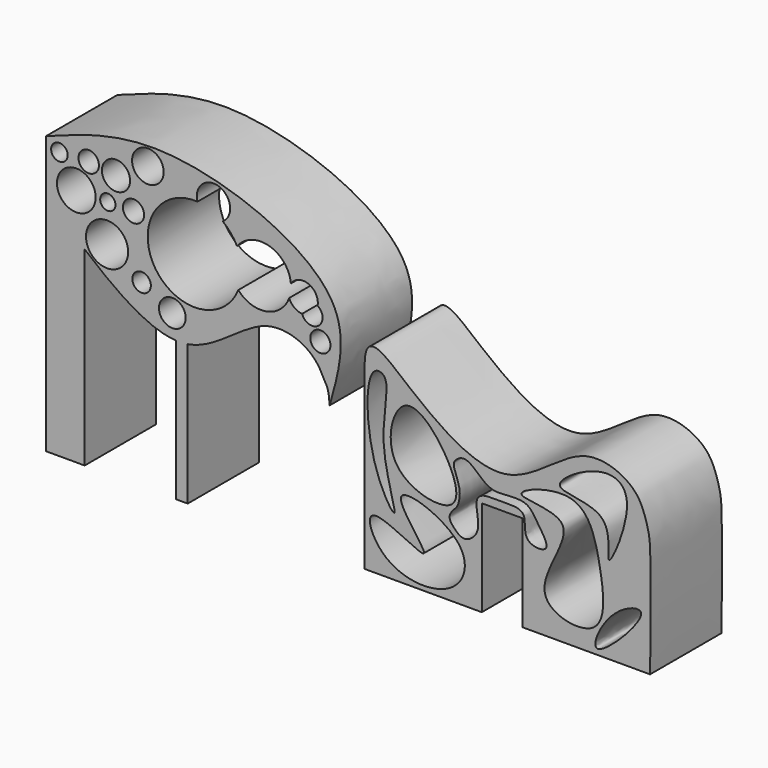
from build123d import *

# Parameters (mm, degrees)
F1_DEPTH = 25
F0_R     = 3.7468792803
F0_R_2   = 2.5930177145
F0_R_3   = 5.9129187482
F0_R_4   = 2.8310435697
F0_R_5   = 5.4292359739
F0_R_6   = 2.1382808776
F0_R_7   = 2.3192836327
F0_R_8   = 3.9494993962
F0_R_9   = 2.868756134
F0_R_10  = 2.9701337928
F0_R_11  = 4.4308880969
F2_DEPTH = 25
F3_DEPTH = 25


# Not quite as in the source:
# - a feature names something its author has since deleted; it is built from what else it names


with BuildPart() as f1:
    # F0 (on Front) → F1 (new body)
    with BuildSketch(Plane.XZ):
        with BuildLine():
            Line((0, 50.3192950504), (0, 0))
            Line((0, 0), (32.8370295465, 0))
            Line((32.8370295465, 0), (32.8370295465, 26.8986206502))
            Line((32.8370295465, 26.8986206502), (44.2832522094, 26.8986206502))
            Line((44.2832522094, 26.8986206502), (44.2832522094, 0))
            Line((44.2832522094, 0), (80.0090666652, 0))
            add(Edge.make_bspline(
                [(0, 50.3192950504), (0, 59.5670401082), (14.3941760892, 46.8630363864), (39.6650361306, 28.0602790595), (59.9123084229, 52.1391667117), (75.1310389197, 45.7993651518), (78.2880633586, 39.9618765746), (79.9116639555, 34.1838305265), (80.0826767357, 30.1384767337), (80.1342161447, 27.1190199724), (80.2397243312, 10.6725007615), (80.0090666652, 0)],
                knots=[0, 0, 0, 0, 0.1048673687, 0.2855122378, 0.4444928656, 0.5600818488, 0.6406896061, 0.7183388135, 0.7795126437, 0.8327719435, 1, 1, 1, 1], degree=3))
        make_face()
        with BuildLine():
            add(Edge.make_bspline(
                [(2.6190045755, 14.0788517892), (5.7735380649, 14.7843920782), (25.3760012063, 1.8985051433), (1.0195787159, 27.2773558636), (30.9160049406, 16.9815187886), (26.8250802338, -0.0133766262), (4.7900411144, 0.6405429526), (0.0622667044, 13.507013962), (2.6190045755, 14.0788517892)],
                knots=[0, 0, 0, 0, 0.1710040186, 0.3333982072, 0.515786692, 0.6683528953, 0.8614018675, 1, 1, 1, 1], degree=3))
        make_face(mode=Mode.SUBTRACT)
        with BuildLine():
            add(Edge.make_bspline(
                [(77.495649457, 14.0632800758), (77.4254563321, 11.254987106), (60.23986575, -6.2126871426), (68.0266170098, 13.1025166472), (77.5437086212, 15.9860355192), (77.495649457, 14.0632800758)],
                knots=[0, 0, 0, 0, 0.4044382334, 0.7230930594, 1, 1, 1, 1], degree=3))
        make_face(mode=Mode.SUBTRACT)
        with BuildLine():
            add(Edge.make_bspline(
                [(2.6190045755, 49.562137574), (-0.0475222277, 46.987181341), (0.6415840322, 26.5382148544), (11.4438679539, 10.8316888041), (2.6835703926, 33.1327162554), (8.1202915155, 49.4531375969), (3.5764535283, 50.4867069972), (2.6190045755, 49.562137574)],
                knots=[0, 0, 0, 0, 0.2688378954, 0.4530209736, 0.6760495052, 0.9034704766, 1, 1, 1, 1], degree=3))
        make_face(mode=Mode.SUBTRACT)
        with BuildLine():
            add(Edge.make_bspline(
                [(8.7999636307, 28.9589390159), (12.0139225942, 23.5678839806), (28.0971888261, 19.9564866654), (24.5008453549, 35.1521631992), (10.0868025916, 51.0773257342), (5.6723666995, 34.205131446), (8.7999636307, 28.9589390159)],
                knots=[0, 0, 0, 0, 0.2663190833, 0.4836403085, 0.7408371553, 1, 1, 1, 1], degree=3))
        make_face(mode=Mode.SUBTRACT)
        with BuildLine():
            add(Edge.make_bspline(
                [(44.0328940749, 32.6909832656), (44.6699120983, 31.4855753989), (64.5626106916, 32.7205472665), (41.987037479, 7.8414458788), (68.6716391837, 2.0469439032), (66.2754723671, 22.6254610166), (61.5480065133, 40.9361936385), (43.3486768569, 33.9857045871), (44.0328940749, 32.6909832656)],
                knots=[0, 0, 0, 0, 0.1476628231, 0.335829375, 0.4950636606, 0.6671411211, 0.8413962521, 1, 1, 1, 1], degree=3))
        make_face(mode=Mode.SUBTRACT)
        with BuildLine():
            add(Edge.make_bspline(
                [(25.0720456243, 18.272837624), (25.8875038676, 17.4027869609), (27.9100110865, 15.6813861052), (31.6300578474, 18.4104435466), (32.07612217, 22.161475039), (30.8199667761, 26.9244646071), (32.7061778665, 29.1536475996), (36.4478146426, 29.12185021), (40.1557735248, 29.173844897), (45.9982486225, 28.9866748309), (43.6693515523, 20.8857068322), (53.1792420497, 20.403362512), (48.3193055137, 27.2157493364), (45.9329611974, 31.2956808101), (40.6584975804, 31.2835436037), (35.4657767382, 30.6005737382), (31.5530871062, 34.0566001583), (28.0340849021, 37.1593977156), (24.4911243904, 34.7510580977), (25.4130809672, 32.1880830646), (26.4885455649, 29.2596642376), (26.8044725158, 27.0026681032), (26.2209382301, 23.9876310328), (25.157328577, 23.0349735937), (23.1635004753, 20.652120897), (24.3363979719, 19.0577346226), (25.0720456243, 18.272837624)],
                knots=[0, 0, 0, 0, 0.0397320435, 0.081232492, 0.1232182551, 0.1701380523, 0.2032798553, 0.2435113911, 0.2876245222, 0.3323792652, 0.3851126704, 0.4336975099, 0.4855691297, 0.5337493517, 0.5807275633, 0.629504686, 0.6783064578, 0.7229409921, 0.7611116883, 0.7945605394, 0.8328380067, 0.8662782619, 0.9027107661, 0.9292506183, 0.9641566141, 1, 1, 1, 1], degree=3))
        make_face(mode=Mode.SUBTRACT)
        with BuildLine():
            add(Edge.make_bspline(
                [(54.8071935773, 38.2395535707), (55.6159599566, 36.4911262021), (70.9861496935, 38.0254487245), (65.9692079193, 16.4864759001), (77.2526212543, 42.3288430166), (66.6630938588, 48.1872312905), (53.9799848043, 40.0278505318), (54.8071935773, 38.2395535707)],
                knots=[0, 0, 0, 0, 0.2055194821, 0.3826390649, 0.6171099844, 0.7897940333, 1, 1, 1, 1], degree=3))
        make_face(mode=Mode.SUBTRACT)
    extrude(amount=F1_DEPTH)


with BuildPart() as f2:
    # F0 (on Front) → F2 (new body)
    with BuildSketch(Plane.XZ):
        with BuildLine():
            Line((-89.300006628, 77.7801488219), (-89.300006628, 53.369268775))
            add(Edge.make_bspline(
                [(-89.300006628, 53.369268775), (-89.300006628, 62.82215087), (-84.0126453614, 58.0148248406), (-78.4782001296, 53.369268775)],
                knots=[0, 0, 0, 0, 0.107193577, 0.107193577, 0.107193577, 0.107193577], degree=3))
            add(Edge.make_bspline(
                [(-78.4782001296, 53.369268775), (-70.0545704822, 46.2985612037), (-61.0585470584, 39.6026093166), (-52.8108254075, 39.1713934549)],
                knots=[0.107193577, 0.107193577, 0.107193577, 0.107193577, 0.2703461524, 0.2703461524, 0.2703461524, 0.2703461524], degree=3))
            add(Edge.make_bspline(
                [(-52.8108254075, 39.1713934549), (-51.7239820399, 39.1145699928), (-50.6501326676, 39.1665314523), (-49.5922993401, 39.3407554389)],
                knots=[0.2703461524, 0.2703461524, 0.2703461524, 0.2703461524, 0.29184558, 0.29184558, 0.29184558, 0.29184558], degree=3))
            add(Edge.make_bspline(
                [(-49.5922993401, 39.3407554389), (-41.596480456, 40.657658023), (-29.3675509948, 54.996079558), (-17.654106763, 50.5730889301), (-14.8029311421, 47.9888351508)],
                knots=[0.29184558, 0.29184558, 0.29184558, 0.29184558, 0.4543527773, 0.5725057998, 0.5725057998, 0.5725057998, 0.5725057998], degree=3))
            add(Edge.make_bspline(
                [(-14.8029311421, 47.9888351508), (-12.8146199192, 46.1866659843), (-10.9129551381, 41.9942429453), (-10.0965067426, 41.0729792704), (-9.7952308133, 37.1719561517)],
                knots=[0.5725057998, 0.5725057998, 0.5725057998, 0.5725057998, 0.6549016294, 0.7329200043, 0.7329200043, 0.7329200043, 0.7329200043], degree=3))
            add(Edge.make_bspline(
                [(-89.300006628, 77.7801488219), (-78.9134210308, 81.696581655), (-56.2566339838, 90.2482278427), (-0.690429825, 68.5155712372), (-7.2166502591, 46.4627534749), (-9.7952308133, 37.1719561517)],
                knots=[0, 0, 0, 0, 0.327733614, 0.7156914248, 1, 1, 1, 1], degree=3))
        make_face()
        with Locations((-53.9055354893, 45.6415861845)):
            Circle(F0_R, mode=Mode.SUBTRACT)
        with Locations((-62.5191554427, 50.4095293581)):
            Circle(F0_R_2, mode=Mode.SUBTRACT)
        with Locations((-72.2038149834, 56.6383376718)):
            Circle(F0_R_3, mode=Mode.SUBTRACT)
        with Locations((-12.4039789662, 52.0625039935)):
            Circle(F0_R_4, mode=Mode.SUBTRACT)
        with BuildLine():
            ThreePointArc((-39.7766612224, 72.8276395151), (-37.4897480211, 70.6611734611), (-35.7822989432, 68.0138795977))
            ThreePointArc((-35.7822989432, 68.0138795977), (-26.7621850313, 71.013252374), (-20.6690978996, 63.7171588136))
            ThreePointArc((-20.6690978996, 63.7171588136), (-16.0399302882, 65.3388441781), (-13.1267671338, 61.3926388323))
            ThreePointArc((-13.1267671338, 61.3926388323), (-13.1440578564, 61.0151463046), (-13.195785223, 60.6408150915))
            ThreePointArc((-13.195785223, 60.6408150915), (-12.1626803516, 59.5720114752), (-11.7860830002, 58.1340193748))
            ThreePointArc((-11.7860830002, 58.1340193748), (-14.283917234, 55.2328793039), (-17.523967202, 57.2719638474))
            ThreePointArc((-17.523967202, 57.2719638474), (-19.7394015452, 58.0933824806), (-21.1417928127, 59.9950072158))
            ThreePointArc((-21.1417928127, 59.9950072158), (-27.5133197329, 54.5959463003), (-35.4090635434, 57.3168733014))
            ThreePointArc((-35.4090635434, 57.3168733014), (-58.769987473, 55.2004539015), (-46.8475612525, 75.4011407942))
            ThreePointArc((-46.8475612525, 75.4011407942), (-43.0285365362, 81.3305694971), (-37.6998727989, 76.7101347446))
            ThreePointArc((-37.6998727989, 76.7101347446), (-38.2516892278, 74.5086114445), (-39.7766612224, 72.8276395151))
        make_face(mode=Mode.SUBTRACT)
        with Locations((-80.8265134692, 67.1438798308)):
            Circle(F0_R_5, mode=Mode.SUBTRACT)
        with Locations((-71.9953626394, 67.101366818)):
            Circle(F0_R_6, mode=Mode.SUBTRACT)
        with Locations((-85.5638608336, 75.0116631389)):
            Circle(F0_R_7, mode=Mode.SUBTRACT)
        with Locations((-69.7007253766, 74.4175761938)):
            Circle(F0_R_8, mode=Mode.SUBTRACT)
        with Locations((-77.3520767689, 75.3619447351)):
            Circle(F0_R_9, mode=Mode.SUBTRACT)
        with Locations((-64.7956952453, 67.2250688076)):
            Circle(F0_R_10, mode=Mode.SUBTRACT)
        with Locations((-60.7653521001, 79.606577754)):
            Circle(F0_R_11, mode=Mode.SUBTRACT)
    extrude(amount=F2_DEPTH)

    # F0 (on Front) → F3 (join)
    with BuildSketch(Plane.XZ):
        with BuildLine():
            add(Edge.make_bspline(
                [(-52.8108254075, 39.1713934549), (-51.7239820399, 39.1145699928), (-50.6501326676, 39.1665314523), (-49.5922993401, 39.3407554389)],
                knots=[0.2703461524, 0.2703461524, 0.2703461524, 0.2703461524, 0.29184558, 0.29184558, 0.29184558, 0.29184558], degree=3))
            Line((-52.8108254075, 39.1713934549), (-52.8108254075, 0))
            Line((-52.8108254075, 0), (-49.5922993401, 0))
            Line((-49.5922993401, 0), (-49.5922993401, 39.3407554389))
        make_face()
        with BuildLine():
            add(Edge.make_bspline(
                [(-89.300006628, 53.369268775), (-89.300006628, 62.82215087), (-84.0126453614, 58.0148248406), (-78.4782001296, 53.369268775)],
                knots=[0, 0, 0, 0, 0.107193577, 0.107193577, 0.107193577, 0.107193577], degree=3))
            Line((-89.300006628, 53.369268775), (-89.300006628, 0))
            Line((-89.300006628, 0), (-78.4782001296, 0))
            Line((-78.4782001296, 0), (-78.4782001296, 53.369268775))
        make_face()
    extrude(amount=F3_DEPTH)


solid = Compound([f1.part, f2.part])
